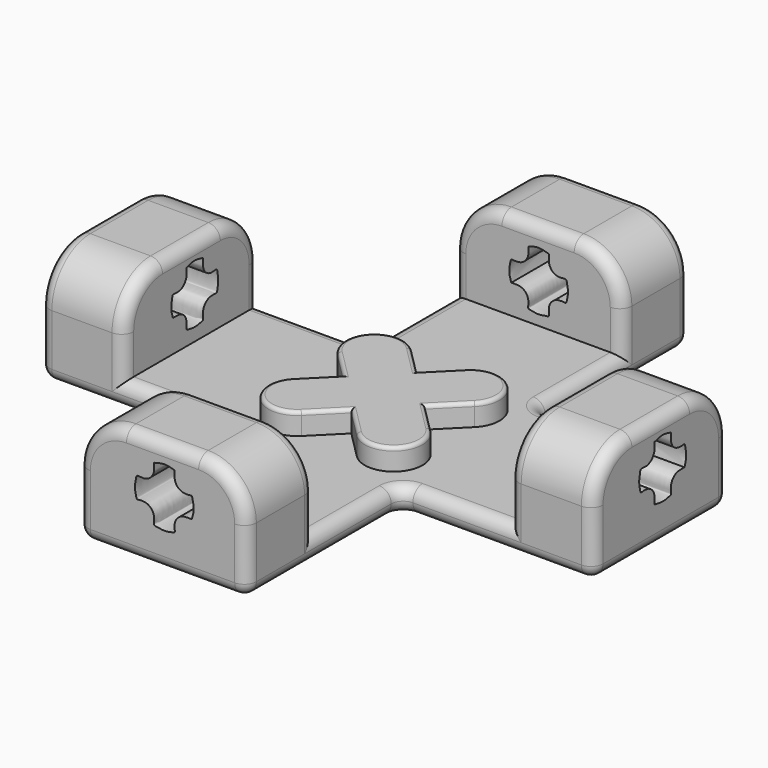
from build123d import *

# Parameters (mm, degrees)
F1_DEPTH  = 1.8
F2_W      = 14
F2_H      = 7
F2_W_2    = 7
F2_H_2    = 14
F3_DEPTH  = 2
F4_W      = 14
F4_H      = 6.9959031225
F4_W_2    = 7
F4_H_2    = 14
F4_H_3    = 7.0040968775
F5_DEPTH  = 7.3
F6_R      = 4
F7_R      = 1
F8_R      = 1
F9_R      = 0.99999
F10_R     = 0.3
F12_DEPTH = 11.1
F14_DEPTH = 8.3
F16_DEPTH = 9.8
F18_DEPTH = 12.3


# Not quite as in the source:
# - a fillet or chamfer is up to 0.001 mm smaller than in the source, because OpenCascade refuses the exact size


with BuildPart() as f1:
    # F0 (on Top) → F1 (new body)
    with BuildSketch(Plane.XY):
        with BuildLine():
            Line((4, -0.6058874503), (1.6970562748, 1.6970562748))
            ThreePointArc((1.6970562748, 1.6970562748), (-1.6970562748, 1.6970562748), (-1.6970562748, -1.6970562748))
            Line((-1.6970562748, -1.6970562748), (0.6058874503, -4))
            Line((0.6058874503, -4), (-1.6970562748, -6.3029437252))
            ThreePointArc((-1.6970562748, -6.3029437252), (-1.6970562748, -9.6970562748), (1.6970562748, -9.6970562748))
            Line((1.6970562748, -9.6970562748), (4, -7.3941125497))
            Line((4, -7.3941125497), (6.3029437252, -9.6970562748))
            ThreePointArc((6.3029437252, -9.6970562748), (9.6970562748, -9.6970562748), (9.6970562748, -6.3029437252))
            Line((9.6970562748, -6.3029437252), (7.3941125497, -4))
            Line((7.3941125497, -4), (9.6970562748, -1.6970562748))
            ThreePointArc((9.6970562748, -1.6970562748), (9.6970562748, 1.6970562748), (6.3029437252, 1.6970562748))
            Line((6.3029437252, 1.6970562748), (4, -0.6058874503))
        make_face()
    extrude(amount=F1_DEPTH)

    # F2 (on Top) → F3 (join)
    with BuildSketch(Plane.XY):
        Polygon((-2.9999892929, 11.9958924155), (-2.9999892929, 2.9999892929), (-11.9999892929, 2.9999892929), (-11.9999892929, -11.0000107071), (-2.9999892929, -11.0000107071), (-2.9999892929, -20.0041075845), (11.0000107071, -20.0041075845), (11.0000107071, -11.0000107071), (20.0000107071, -11.0000107071), (20.0000107071, 2.9999892929), (11.0000107071, 2.9999892929), (11.0000107071, 11.9958924155), align=None)
        with Locations((4.0000107071, 15.4958924155)):
            Rectangle(F2_W, F2_H)
        with Locations((23.5000107071, -4.0000107071)):
            Rectangle(F2_W_2, F2_H_2)
        with Locations((4.0000107071, -23.5041075845)):
            Rectangle(F2_W, F2_H)
        with Locations((-15.4999892929, -4.0000107071)):
            Rectangle(F2_W_2, F2_H_2)
    extrude(amount=-F3_DEPTH)

    # F4 (on Top) → F5 (join)
    with BuildSketch(Plane.XY):
        with Locations((4.0000107071, 15.4979408542)):
            Rectangle(F4_W, F4_H)
        with Locations((23.5000107071, -4.0000107071)):
            Rectangle(F4_W_2, F4_H_2)
        with Locations((4.0000107071, -23.5020591458)):
            Rectangle(F4_W, F4_H_3)
        with Locations((-15.4999892929, -4.0000107071)):
            Rectangle(F4_W_2, F4_H_2)
    extrude(amount=F5_DEPTH)

    # F6
    f6_edges = [f1.edges().sort_by_distance(p)[0] for p in [
        (-15.499989, -11.000011, 7.3),
        (-15.499989, 2.999989, 7.3),
        (-2.999989, 15.497941, 7.3),
        (11.000011, 15.497941, 7.3),
        (23.500011, 2.999989, 7.3),
        (23.500011, -11.000011, 7.3),
        (11.000011, -23.502059, 7.3),
        (-2.999989, -23.502059, 7.3),
    ]]
    fillet(f6_edges, radius=F6_R)

    # F7
    f7_edges = [f1.edges().sort_by_distance(p)[0] for p in [
        (11.000011, 2.999989, -1),
        (11.000011, -11.000011, -1),
        (-2.999989, -11.000011, -1),
        (-2.999989, 2.999989, -1),
    ]]
    fillet(f7_edges, radius=F7_R)

    # F8
    f8_edges = [f1.edges().sort_by_distance(p)[0] for p in [
        (4.000011, 11.999989, 7.3),
        (-2.999989, 7.999989, 0),
        (11.000011, 7.999989, 0),
        (16.000011, 2.999989, 0),
        (16.000011, -11.000011, 0),
        (11.000011, -16.000011, 0),
        (-2.999989, -16.000011, 0),
        (-7.999989, -11.000011, 0),
        (-11.999989, -11.000011, 1.65),
        (-11.999989, -9.828438, 6.128427),
        (-7.999989, 2.999989, 0),
        (-1.828416, -20.000011, 6.128427),
        (20.000011, -4.000011, 7.3),
    ]]
    fillet(f8_edges, radius=F8_R)

    # F9 (radius 1 in the source; OpenCascade refuses exactly that, so slightly less here)
    f9_edges = [f1.edges().sort_by_distance(p)[0] for p in [
        (-18.999989, -4.000011, -2),
        (-11.499989, -11.000011, -2),
        (-2.999989, -19.502059, -2),
        (4.000011, -27.004108, -2),
        (11.000011, -19.502059, -2),
        (19.500011, -11.000011, -2),
        (27.000011, -4.000011, -2),
        (19.500011, 2.999989, -2),
        (11.000011, 11.497941, -2),
        (4.000011, 18.995892, -2),
        (-2.999989, 11.497941, -2),
        (-11.499989, 2.999989, -2),
        (11.000011, -27.004108, 0.65),
        (-18.999989, -11.000011, 0.65),
        (11.000011, 18.995892, 0.65),
        (27.000011, -11.000011, 0.65),
        (9.828438, 18.995892, 6.128427),
        (4.000011, 18.995892, 7.3),
        (-1.828416, 18.995892, 6.128427),
        (-2.999989, 18.995892, 0.65),
        (27.000011, -9.828438, 6.128427),
    ]]
    fillet(f9_edges, radius=F9_R)

    # F10
    f10_edges = [f1.edges().sort_by_distance(p)[0] for p in [
        (-0.545584, -5.151472, 1.8),
        (-0.545584, -2.848528, 1.8),
        (5.151472, 0.545584, 1.8),
        (8.545584, -5.151472, 1.8),
    ]]
    fillet(f10_edges, radius=F10_R)

    # F11 (on face) → F12 (cut)
    with BuildSketch(Plane.XZ.offset(27.0041075845)):
        with BuildLine():
            add(Edge.make_bspline(
                [(3.2999345567, 5.6037250354), (3.5975526746, 5.687586009), (4.1816535074, 5.8550049268), (4.7306632188, 5.685472247), (4.99993539, 5.6037250354)],
                knots=[0, 0, 0, 0, 0.5095712537, 1, 1, 1, 1], degree=3))
            add(Edge.make_bspline(
                [(3.2999345567, 5.6037250354), (3.2997914577, 5.5046207932), (3.2995172318, 5.3147037295), (3.3013678423, 5.0579319697), (3.285142881, 4.8691711493), (3.1132152772, 4.5109370035), (2.9103884839, 4.3399213093), (2.6332595755, 4.2046464216), (2.3401893985, 4.152558247), (1.8063008396, 4.2848611379), (1.8028826955, 3.8836441954), (1.7190545507, 3.6225455659), (1.7057796695, 3.2865589672), (1.7304193555, 2.9964102571), (1.8037103792, 2.7530704225), (1.8385097046, 2.422824589), (2.085853781, 2.500540438), (2.3861098643, 2.4860762542), (2.6380285172, 2.4540894493), (2.8278573971, 2.3781123023), (3.0562738656, 2.1977796206), (3.1587343758, 2.056189962), (3.2569892854, 1.8763615175), (3.3031584367, 1.6178673329), (3.3160078463, 1.3931150125), (3.2239329679, 1.000952697), (3.5759092492, 0.9936268881), (3.8992705822, 0.9081798955), (4.1858347415, 0.9067191821), (4.449198525, 0.9117858339), (4.7992494383, 1.0119655112), (5.0600825983, 1.0125224534), (4.98740033, 1.3996974833), (4.9897909642, 1.647397314), (5.0917665392, 1.9978521743), (5.2336839413, 2.1863371986), (5.5038025959, 2.4191094542), (5.9300956535, 2.5007364234), (6.2533076094, 2.4887699322), (6.42106539, 2.4825589243)],
                knots=[0, 0, 0, 0, 0.0273605905, 0.0524320947, 0.0745076412, 0.1056108167, 0.1318649214, 0.158948127, 0.1874687016, 0.220995097, 0.2482860623, 0.2755720453, 0.3045111481, 0.3315301836, 0.3578655515, 0.3837385363, 0.4059679792, 0.434252013, 0.4594532962, 0.4822711791, 0.5090972104, 0.530231005, 0.5527300135, 0.5781274322, 0.6031996615, 0.6315546276, 0.6576667534, 0.6876672756, 0.714256594, 0.7402463844, 0.7710533559, 0.7932728015, 0.8216277676, 0.8482190477, 0.8777914221, 0.9023565188, 0.9315770045, 0.9644861842, 1, 1, 1, 1], degree=3))
            add(Edge.make_bspline(
                [(4.99993539, 5.6037250354), (4.9903855992, 5.410602556), (4.9727074583, 5.0432135196), (5.1083607047, 4.5888663629), (5.4523542561, 4.2786253369), (5.7951388392, 4.1733246286), (6.2046649316, 4.1639772963), (6.4586618911, 4.2377288636), (6.4965806342, 3.9160063414), (6.5923645303, 3.5592725409), (6.5906724356, 3.213239591), (6.5541039775, 2.8899520136), (6.4669974864, 2.6249335584), (6.42106539, 2.4825589243)],
                knots=[0, 0, 0, 0, 0.1117445823, 0.2125923647, 0.3107430927, 0.4000660841, 0.4960442665, 0.5626441507, 0.6379036869, 0.7311412958, 0.8178947498, 0.9022950941, 1, 1, 1, 1], degree=3))
        make_face()
    extrude(amount=-F12_DEPTH, mode=Mode.SUBTRACT)

    # F13 (on face) → F14 (cut)
    with BuildSketch(Plane.YZ.offset(27.0000107071)):
        with BuildLine():
            add(Edge.make_bspline(
                [(-4.6549346298, 5.7423317951), (-4.3573165119, 5.8261927687), (-3.7732156791, 5.9936116865), (-3.2242059677, 5.8240790068), (-2.9549337965, 5.7423317951)],
                knots=[0, 0, 0, 0, 0.5095712537, 1, 1, 1, 1], degree=3))
            add(Edge.make_bspline(
                [(-4.6549346298, 5.7423317951), (-4.6550777288, 5.6432275529), (-4.6553519547, 5.4533104892), (-4.6535013442, 5.1965387294), (-4.6697263055, 5.0077779091), (-4.8416539093, 4.6495437632), (-5.0444807026, 4.478528069), (-5.321609611, 4.3432531813), (-5.614679788, 4.2911650067), (-6.1485683469, 4.4234678977), (-6.151986491, 4.0222509551), (-6.2358146358, 3.7611523257), (-6.2490895171, 3.425165727), (-6.224449831, 3.1350170168), (-6.1511588073, 2.8916771822), (-6.1163594819, 2.5614313487), (-5.8690154055, 2.6391471977), (-5.5687593222, 2.6246830139), (-5.3168406693, 2.5926962091), (-5.1270117894, 2.516719062), (-4.8985953209, 2.3363863804), (-4.7961348107, 2.1947967217), (-4.6978799011, 2.0149682772), (-4.6517107498, 1.7564740926), (-4.6388613402, 1.5317217722), (-4.7309362186, 1.1395594567), (-4.3789599373, 1.1322336478), (-4.0555986043, 1.0467866552), (-3.769034445, 1.0453259418), (-3.5056706615, 1.0503925936), (-3.1556197482, 1.1505722709), (-2.8947865882, 1.1511292131), (-2.9674688565, 1.5383042431), (-2.9650782224, 1.7860040737), (-2.8631026473, 2.136458934), (-2.7211852453, 2.3249439584), (-2.4510665906, 2.5577162139), (-2.024773533, 2.6393431832), (-1.7015615771, 2.6273766919), (-1.5338037965, 2.621165684)],
                knots=[0, 0, 0, 0, 0.0273605905, 0.0524320947, 0.0745076412, 0.1056108167, 0.1318649214, 0.158948127, 0.1874687016, 0.220995097, 0.2482860623, 0.2755720453, 0.3045111481, 0.3315301836, 0.3578655515, 0.3837385363, 0.4059679792, 0.434252013, 0.4594532962, 0.4822711791, 0.5090972104, 0.530231005, 0.5527300135, 0.5781274322, 0.6031996615, 0.6315546276, 0.6576667534, 0.6876672756, 0.714256594, 0.7402463844, 0.7710533559, 0.7932728015, 0.8216277676, 0.8482190477, 0.8777914221, 0.9023565188, 0.9315770045, 0.9644861842, 1, 1, 1, 1], degree=3))
            add(Edge.make_bspline(
                [(-2.9549337965, 5.7423317951), (-2.9644835873, 5.5492093157), (-2.9821617282, 5.1818202794), (-2.8465084818, 4.7274731226), (-2.5025149304, 4.4172320966), (-2.1597303473, 4.3119313883), (-1.7502042549, 4.302584056), (-1.4962072954, 4.3763356233), (-1.4582885523, 4.0546131012), (-1.3625046562, 3.6978793007), (-1.3641967509, 3.3518463508), (-1.400765209, 3.0285587733), (-1.4878717002, 2.7635403182), (-1.5338037965, 2.621165684)],
                knots=[0, 0, 0, 0, 0.1117445823, 0.2125923647, 0.3107430927, 0.4000660841, 0.4960442665, 0.5626441507, 0.6379036869, 0.7311412958, 0.8178947498, 0.9022950941, 1, 1, 1, 1], degree=3))
        make_face()
    extrude(amount=-F14_DEPTH, mode=Mode.SUBTRACT)

    # F15 (on face) → F16 (cut)
    with BuildSketch(Plane(origin=(0, 18.9958924155, 0), x_dir=(-1, 0, 0), z_dir=(0, 1, 0))):
        with BuildLine():
            add(Edge.make_bspline(
                [(-4.8975730315, 5.5423315528), (-4.5999549136, 5.6261925264), (-4.0158540808, 5.7936114442), (-3.4668443694, 5.6240787644), (-3.1975721982, 5.5423315528)],
                knots=[0, 0, 0, 0, 0.5095712537, 1, 1, 1, 1], degree=3))
            add(Edge.make_bspline(
                [(-4.8975730315, 5.5423315528), (-4.8977161305, 5.4432273106), (-4.8979903564, 5.2533102469), (-4.8961397459, 4.9965384871), (-4.9123647072, 4.8077776667), (-5.084292311, 4.4495435209), (-5.2871191043, 4.2785278267), (-5.5642480127, 4.143252939), (-5.8573181897, 4.0911647644), (-6.3912067486, 4.2234676553), (-6.3946248927, 3.8222507128), (-6.4784530375, 3.5611520833), (-6.4917279187, 3.2251654846), (-6.4670882327, 2.9350167745), (-6.393797209, 2.6916769399), (-6.3589978836, 2.3614311064), (-6.1116538072, 2.4391469554), (-5.8113977239, 2.4246827716), (-5.559479071, 2.3926959667), (-5.3696501911, 2.3167188197), (-5.1412337226, 2.136386138), (-5.0387732124, 1.9947964794), (-4.9405183028, 1.8149680349), (-4.8943491515, 1.5564738503), (-4.8814997419, 1.3317215299), (-4.9735746203, 0.9395592144), (-4.6215983389, 0.9322334055), (-4.298237006, 0.8467864129), (-4.0116728467, 0.8453256995), (-3.7483090631, 0.8503923513), (-3.3982581499, 0.9505720286), (-3.1374249899, 0.9511289708), (-3.2101072582, 1.3383040007), (-3.207716624, 1.5860038314), (-3.105741049, 1.9364586917), (-2.9638236469, 2.124943716), (-2.6937049923, 2.3577159716), (-2.2674119346, 2.4393429408), (-1.9441999788, 2.4273764496), (-1.7764421982, 2.4211654417)],
                knots=[0, 0, 0, 0, 0.0273605905, 0.0524320947, 0.0745076412, 0.1056108167, 0.1318649214, 0.158948127, 0.1874687016, 0.220995097, 0.2482860623, 0.2755720453, 0.3045111481, 0.3315301836, 0.3578655515, 0.3837385363, 0.4059679792, 0.434252013, 0.4594532962, 0.4822711791, 0.5090972104, 0.530231005, 0.5527300135, 0.5781274322, 0.6031996615, 0.6315546276, 0.6576667534, 0.6876672756, 0.714256594, 0.7402463844, 0.7710533559, 0.7932728015, 0.8216277676, 0.8482190477, 0.8777914221, 0.9023565188, 0.9315770045, 0.9644861842, 1, 1, 1, 1], degree=3))
            add(Edge.make_bspline(
                [(-3.1975721982, 5.5423315528), (-3.207121989, 5.3492090733), (-3.2248001299, 4.981820037), (-3.0891468835, 4.5274728803), (-2.7451533321, 4.2172318542), (-2.402368749, 4.111931146), (-1.9928426566, 4.1025838136), (-1.7388456971, 4.176335381), (-1.700926954, 3.8546128588), (-1.6051430579, 3.4978790583), (-1.6068351526, 3.1518461084), (-1.6434036107, 2.828558531), (-1.7305101018, 2.5635400758), (-1.7764421982, 2.4211654417)],
                knots=[0, 0, 0, 0, 0.1117445823, 0.2125923647, 0.3107430927, 0.4000660841, 0.4960442665, 0.5626441507, 0.6379036869, 0.7311412958, 0.8178947498, 0.9022950941, 1, 1, 1, 1], degree=3))
        make_face()
    extrude(amount=-F16_DEPTH, mode=Mode.SUBTRACT)

    # F17 (on face) → F18 (cut)
    with BuildSketch(Plane(origin=(-18.9999892929, 0, 0), x_dir=(0, -1, 0), z_dir=(-1, 0, 0))):
        with BuildLine():
            add(Edge.make_bspline(
                [(2.8033523837, 5.7632265992), (3.1009705015, 5.8470875727), (3.6850713343, 6.0145064905), (4.2340810457, 5.8449738108), (4.503353217, 5.7632265992)],
                knots=[0, 0, 0, 0, 0.5095712537, 1, 1, 1, 1], degree=3))
            add(Edge.make_bspline(
                [(2.8033523837, 5.7632265992), (2.8032092846, 5.6641223569), (2.8029350588, 5.4742052932), (2.8047856693, 5.2174335335), (2.788560708, 5.0286727131), (2.6166331042, 4.6704385673), (2.4138063109, 4.499422873), (2.1366774025, 4.3641479854), (1.8436072255, 4.3120598108), (1.3097186665, 4.4443627017), (1.3063005224, 4.0431457591), (1.2224723776, 3.7820471297), (1.2091974964, 3.446060531), (1.2338371825, 3.1559118208), (1.3071282061, 2.9125719863), (1.3419275316, 2.5823261527), (1.5892716079, 2.6600420018), (1.8895276912, 2.645577818), (2.1414463442, 2.6135910131), (2.3312752241, 2.5376138661), (2.5596916926, 2.3572811844), (2.6621522027, 2.2156915257), (2.7604071124, 2.0358630813), (2.8065762636, 1.7773688966), (2.8194256732, 1.5526165763), (2.7273507948, 1.1604542607), (3.0793270762, 1.1531284518), (3.4026884092, 1.0676814592), (3.6892525685, 1.0662207458), (3.952616352, 1.0712873977), (4.3026672652, 1.1714670749), (4.5635004253, 1.1720240172), (4.490818157, 1.5591990471), (4.4932087911, 1.8068988778), (4.5951843661, 2.157353738), (4.7371017682, 2.3458387624), (5.0072204228, 2.578611018), (5.4335134805, 2.6602379872), (5.7567254363, 2.648271496), (5.924483217, 2.6420604881)],
                knots=[0, 0, 0, 0, 0.0273605905, 0.0524320947, 0.0745076412, 0.1056108167, 0.1318649214, 0.158948127, 0.1874687016, 0.220995097, 0.2482860623, 0.2755720453, 0.3045111481, 0.3315301836, 0.3578655515, 0.3837385363, 0.4059679792, 0.434252013, 0.4594532962, 0.4822711791, 0.5090972104, 0.530231005, 0.5527300135, 0.5781274322, 0.6031996615, 0.6315546276, 0.6576667534, 0.6876672756, 0.714256594, 0.7402463844, 0.7710533559, 0.7932728015, 0.8216277676, 0.8482190477, 0.8777914221, 0.9023565188, 0.9315770045, 0.9644861842, 1, 1, 1, 1], degree=3))
            add(Edge.make_bspline(
                [(4.503353217, 5.7632265992), (4.4938034262, 5.5701041197), (4.4761252853, 5.2027150834), (4.6117785316, 4.7483679267), (4.9557720831, 4.4381269006), (5.2985566662, 4.3328261923), (5.7080827586, 4.32347886), (5.962079718, 4.3972304274), (5.9999984612, 4.0755079052), (6.0957823573, 3.7187741047), (6.0940902626, 3.3727411548), (6.0575218044, 3.0494535773), (5.9704153133, 2.7844351222), (5.924483217, 2.6420604881)],
                knots=[0, 0, 0, 0, 0.1117445823, 0.2125923647, 0.3107430927, 0.4000660841, 0.4960442665, 0.5626441507, 0.6379036869, 0.7311412958, 0.8178947498, 0.9022950941, 1, 1, 1, 1], degree=3))
        make_face()
    extrude(amount=-F18_DEPTH, mode=Mode.SUBTRACT)


solid = f1.part
